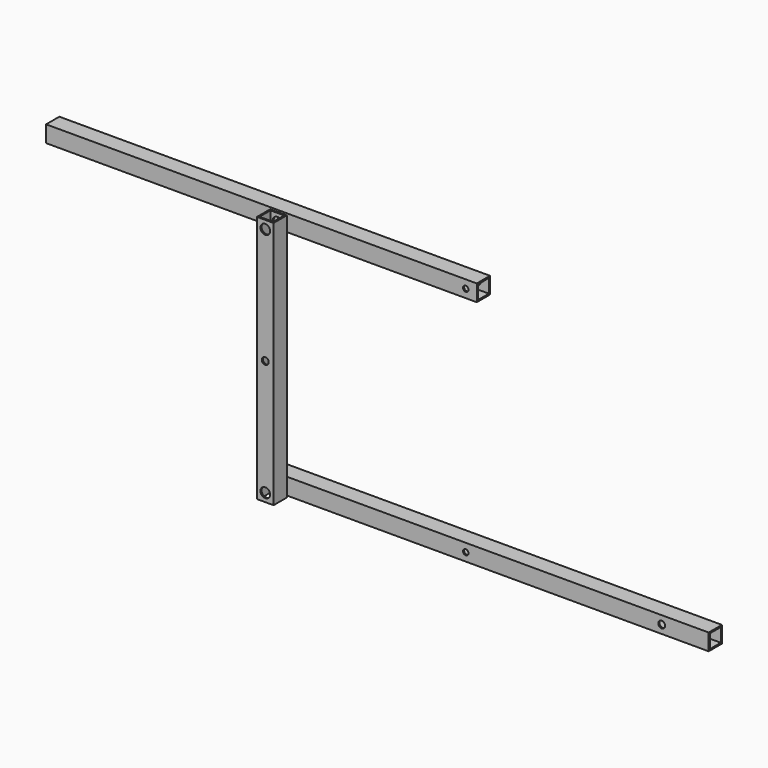
from build123d import *

# Parameters (mm, degrees)
F0_W      = 508
F0_H      = 19.05
F1_DEPTH  = 19.05
F2_T      = -1.6002
F3_R      = 3.175
F4_DEPTH  = 19.051
F7_R      = 5.55625
F8_DEPTH  = 19.05
F9_T      = -1.6002
F10_W     = 495.3
F10_H     = 19.05
F10_R     = 3.175
F11_DEPTH = 19.05
F12_T     = -1.6002
F13_R     = 3.96875
F14_DEPTH = 25.4
F15_R     = 3.9751
F16_DEPTH = 19.051


# Not quite as in the source:
# - a feature names something its author has since deleted; it is built from what else it names


with BuildPart() as f1:
    # F0 (on Front) → F1 (new body)
    with BuildSketch(Plane.XZ):
        with Locations((254, 9.525)):
            Rectangle(F0_W, F0_H)
    extrude(amount=-F1_DEPTH)

    # F2
    f2_openings = [f1.faces().sort_by_distance(p)[0] for p in [
        (508, 9.525, 9.525),
        (0, 9.525, 9.525),
    ]]
    offset(amount=F2_T, openings=f2_openings)

    # F3 (on face) → F4 (cut, through all)
    with BuildSketch(Plane.XZ):
        with Locations((228.6, 9.525)):
            Circle(F3_R)
        with Locations((15.875, 9.525)):
            Circle(F3_R)
    extrude(amount=-F4_DEPTH, mode=Mode.SUBTRACT)

    # F15 (on face) → F16 (cut, through all)
    with BuildSketch(Plane.XZ):
        with Locations((454.025, 9.525)):
            Circle(F15_R)
    extrude(amount=-F16_DEPTH, mode=Mode.SUBTRACT)


with BuildPart() as f8:
    # F7 (on offset) → F8 (new body)
    with BuildSketch(Plane.XZ.offset(3.175)):
        Polygon((25.4, 285.75), (6.35, 285.75), (6.35, 276.225), (6.35, 0), (25.4, 0), (25.4, 276.225), align=None)
        with Locations((15.875, 9.525)):
            Circle(F7_R, mode=Mode.SUBTRACT)
        with Locations((15.875, 276.225)):
            Circle(F7_R, mode=Mode.SUBTRACT)
    extrude(amount=F8_DEPTH)

    # F9
    f9_openings = [f8.faces().sort_by_distance(p)[0] for p in [
        (10.31875, -12.7, 276.225),
        (15.875, -12.7, 0),
        (10.31875, -12.7, 9.525),
        (15.875, -12.7, 285.75),
    ]]
    offset(amount=F9_T, openings=f9_openings)

    # F13 (on face) → F14 (cut)
    with BuildSketch(Plane.XZ.offset(22.225)):
        with Locations((15.875, 142.875)):
            Circle(F13_R)
    extrude(amount=-F14_DEPTH, mode=Mode.SUBTRACT)


with BuildPart() as f11:
    # F10 (on Front) → F11 (new body)
    with BuildSketch(Plane.XZ):
        with Locations((-6.35, 276.225)):
            Rectangle(F10_W, F10_H)
        with Locations((15.875, 276.225)):
            Circle(F10_R, mode=Mode.SUBTRACT)
        with Locations((228.6, 276.225)):
            Circle(F10_R, mode=Mode.SUBTRACT)
    extrude(amount=-F11_DEPTH)

    # F12
    f12_openings = [f11.faces().sort_by_distance(p)[0] for p in [
        (-254, 9.525, 276.225),
        (12.7, 9.525, 276.225),
        (241.3, 9.525, 276.225),
        (225.425, 9.525, 276.225),
    ]]
    offset(amount=F12_T, openings=f12_openings)


solid = Compound([f1.part, f8.part, f11.part])
